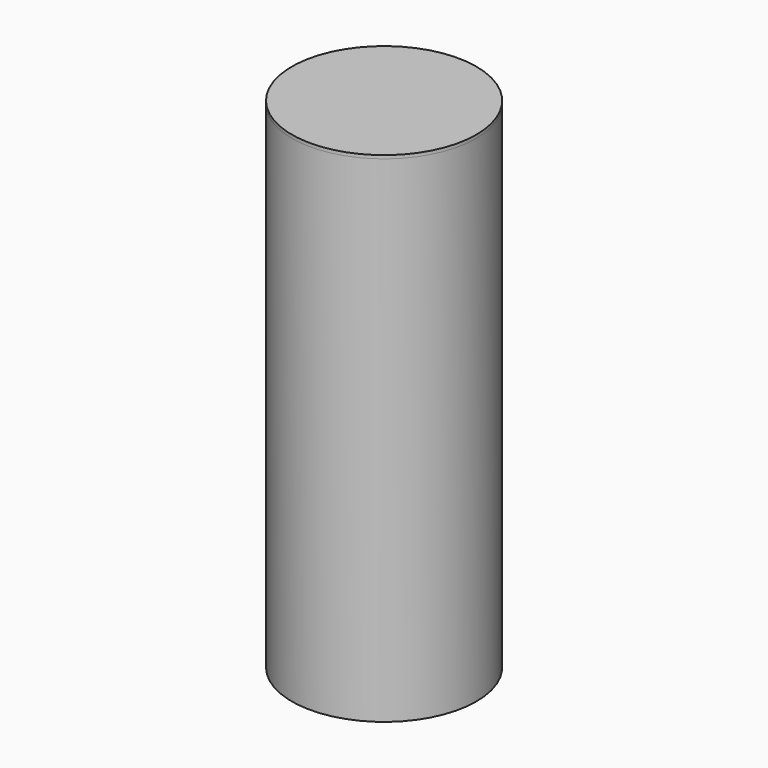
from build123d import *

# Parameters (mm, degrees)
F0_R     = 33.5
F0_R_2   = 32.5
F1_DEPTH = 180
F2_DEPTH = 1.2
F3_R     = 33.5
F3_R_2   = 32.5
F3_R_3   = 31.5
F4_DEPTH = 1.2
F5_DEPTH = 10


with BuildPart() as f1:
    # F0 (on Top) → F1 (new body)
    with BuildSketch(Plane.XY):
        Circle(F0_R)
        Circle(F0_R_2, mode=Mode.SUBTRACT)
    extrude(amount=F1_DEPTH)

    # F0 (on Top) → F2 (join)
    with BuildSketch(Plane.XY):
        Circle(F0_R_2)
    extrude(amount=F2_DEPTH)


with BuildPart() as f4:
    # F3 (on face) → F4 (new body)
    with BuildSketch(Plane.XY.offset(180)):
        Circle(F3_R)
        Circle(F3_R_2, mode=Mode.SUBTRACT)
        Circle(F3_R_2)
        Circle(F3_R_3, mode=Mode.SUBTRACT)
        Circle(F3_R_3)
    extrude(amount=F4_DEPTH)

    # F3 (on face) → F5 (join)
    with BuildSketch(Plane.XY.offset(180)):
        Circle(F3_R_2)
        Circle(F3_R_3, mode=Mode.SUBTRACT)
    extrude(amount=-F5_DEPTH)


solid = Compound([f1.part, f4.part])
